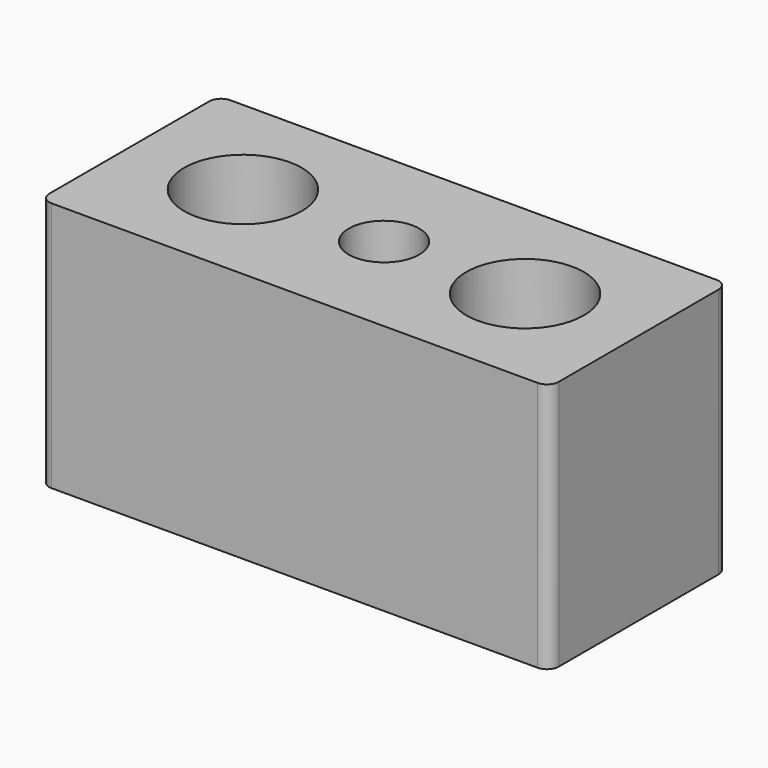
from build123d import *

# Parameters (mm, degrees)
F0_W                 = 65
F0_H                 = 32
F1_DEPTH             = 14.25
F4_D                 = 9
F4_DEPTH             = 40
F4_CBORE_D           = 15
F4_CBORE_DEPTH       = 12
F4_TIP               = 2.7038727856
F4_ON_F3_D           = 9
F4_ON_F3_DEPTH       = 40
F4_ON_F3_CBORE_D     = 15
F4_ON_F3_CBORE_DEPTH = 12
F4_ON_F3_TIP         = 2.7038727856
F5_R                 = 1.5


with BuildPart() as f1:
    # F0 (on Front) → F1 (new body, symmetric)
    with BuildSketch(Plane.XZ):
        Rectangle(F0_W, F0_H)
    extrude(amount=F1_DEPTH, both=True)

    # F4
    with Locations(Plane.XY.offset(16)):
        with Locations((-18, 0), (18, 0)):
            CounterBoreHole(F4_D / 2, F4_CBORE_D / 2, F4_CBORE_DEPTH, depth=F4_DEPTH)
            with Locations((0, 0, -(F4_DEPTH + F4_TIP / 2))):  # 118° drill point
                Cone(0, F4_D / 2, F4_TIP, mode=Mode.SUBTRACT)

    # F4 on F3
    with Locations(Plane(origin=(0, 0, -16), x_dir=(1, 0, 0), z_dir=(0, 0, -1))):
        with Locations((0, 0)):
            CounterBoreHole(F4_ON_F3_D / 2, F4_ON_F3_CBORE_D / 2, F4_ON_F3_CBORE_DEPTH, depth=F4_ON_F3_DEPTH)
            with Locations((0, 0, -(F4_ON_F3_DEPTH + F4_ON_F3_TIP / 2))):  # 118° drill point
                Cone(0, F4_ON_F3_D / 2, F4_ON_F3_TIP, mode=Mode.SUBTRACT)

    # F5
    f5_edges = [f1.edges().sort_by_distance(p)[0] for p in [
        (-32.5, -14.25, 0),
        (32.5, -14.25, 0),
        (32.5, 14.25, 0),
        (-32.5, 14.25, 0),
    ]]
    fillet(f5_edges, radius=F5_R)


solid = f1.part
